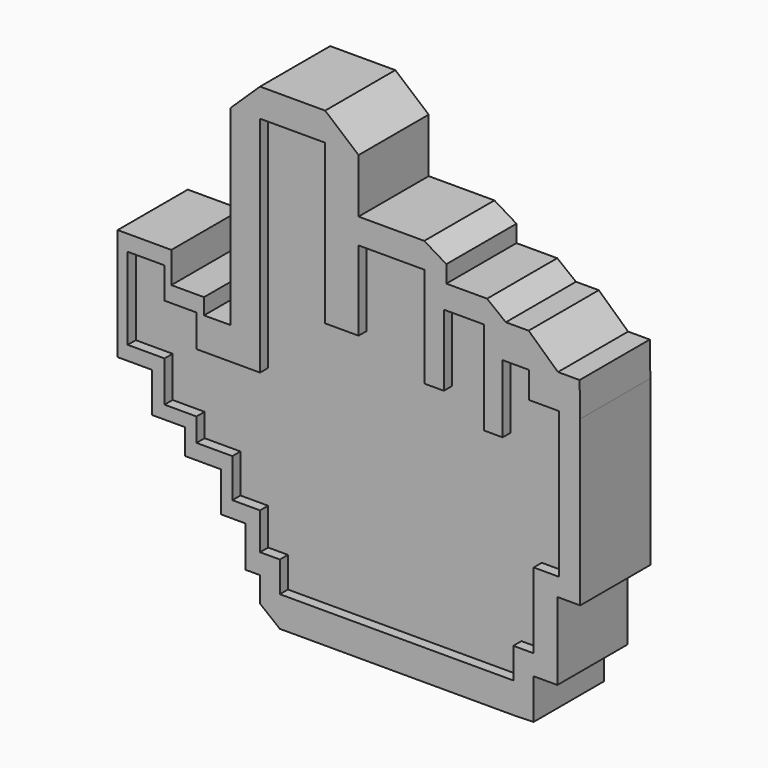
from build123d import *

# Parameters (mm, degrees)
F1_DEPTH = 11.684
F2_DEPTH = 13.208


# Not quite as in the source:
# - a feature names something its author has since deleted; it is built from what else it names


with BuildPart() as f1:
    # F0 (on Front) → F1 (new body)
    with BuildSketch(Plane.XZ):
        Polygon((9.8076034337, -4.2564473115), (0, -4.2564473115), (0, -28.2072033733), (0, -37.9272252321), (-4.4246674515, -37.9272252321), (-9.569064714, -37.9272252321), (-9.569064714, -33.0672143027), (-14.3852122128, -33.0672143027), (-14.3852122128, -28.3846426755), (-19.9310798198, -28.3846426755), (-19.9310798198, -40.7246947289), (-14.3852122128, -40.7246947289), (-14.3852122128, -46.85433954), (-9.569064714, -46.85433954), (-9.569064714, -50.3569915891), (-4.1691423394, -50.3569915891), (-4.1691423394, -56.1947450042), (0, -56.1947450042), (0, -61.7406144738), (2.9821074568, -61.7406144738), (2.9821074568, -66.3378462195), (38.154579699, -66.3378462195), (38.154579699, -61.7406144738), (41.2194021046, -61.7406144738), (41.2194021046, -50.3569915891), (45.0411513448, -50.3569915891), (45.0411513448, -28.3846426755), (40.5284799635, -28.3846426755), (40.5284799635, -24.3923105299), (36.5364998579, -24.3923105299), (36.5364998579, -34.6322879195), (33.7594784796, -34.6322879195), (33.7594784796, -24.3923105299), (33.7594784796, -20.5733645707), (27.6847239584, -20.5733645707), (27.6847239584, -31.3338786364), (24.7341338545, -31.3338786364), (24.7341338545, -20.5733645707), (24.7341338545, -16.2325797137), (14.8409679532, -16.2325797137), (14.8409679532, -28.2087121159), (9.8076034337, -28.2087121159), align=None)
    extrude(amount=F1_DEPTH)

    # F0 (on Front) → F2 (join)
    with BuildSketch(Plane.XZ):
        Polygon((9.8076034337, 0), (0, 0), (-4.4246674515, -4.2564473115), (-4.4246674515, -28.2072033733), (-4.4246674515, -33.0672143027), (-8.441273123, -33.0877043307), (-8.441273123, -30.6703820825), (-13.3577445522, -30.6703820825), (-13.3577445522, -26.0001793504), (-21.4487463236, -26.0001793504), (-21.4487463236, -42.8537763655), (-16.2677373737, -42.8537763655), (-16.2677373737, -48.8393343985), (-11.3371098414, -48.8393343985), (-11.3371098414, -52.6647716761), (-5.9138466604, -52.6647716761), (-5.9138466604, -58.6375892162), (-2.1712374873, -58.6375892162), (-2.1712374873, -64.7857561707), (0, -64.7857561707), (0, -68.5636028647), (2.9821074568, -70.9350779653), (38.154579699, -70.9350779653), (41.2194021046, -70.8393231034), (41.2194021046, -64.7857561707), (44.7839312255, -64.7857561707), (44.7839312255, -61.7406144738), (44.7839312255, -53.1140379608), (48.2247062027, -53.1140379608), (48.2247062027, -50.3569915891), (48.2247062027, -28.3846426755), (48.131018877, -23.2601258904), (44.8739007115, -23.2601258904), (40.4558517039, -19.210241735), (37.0195880532, -19.210241735), (34.1969430447, -17.0012172312), (28.0607584864, -17.0012172312), (28.0607584864, -14.4240194932), (24.7341338545, -12.4151380733), (14.8409679532, -12.4151380733), (14.8409679532, -4.2564473115), align=None)
        Polygon((0, -28.2072033733), (0, -4.2564473115), (9.8076034337, -4.2564473115), (9.8076034337, -28.2087121159), (14.8409679532, -28.2087121159), (14.8409679532, -16.2325797137), (24.7341338545, -16.2325797137), (24.7341338545, -20.5733645707), (24.7341338545, -31.3338786364), (27.6847239584, -31.3338786364), (27.6847239584, -20.5733645707), (33.7594784796, -20.5733645707), (33.7594784796, -24.3923105299), (33.7594784796, -34.6322879195), (36.5364998579, -34.6322879195), (36.5364998579, -24.3923105299), (40.5284799635, -24.3923105299), (40.5284799635, -28.3846426755), (45.0411513448, -28.3846426755), (45.0411513448, -50.3569915891), (41.2194021046, -50.3569915891), (41.2194021046, -61.7406144738), (38.154579699, -61.7406144738), (38.154579699, -66.3378462195), (2.9821074568, -66.3378462195), (2.9821074568, -61.7406144738), (0, -61.7406144738), (0, -56.1947450042), (-4.1691423394, -56.1947450042), (-4.1691423394, -50.3569915891), (-9.569064714, -50.3569915891), (-9.569064714, -46.85433954), (-14.3852122128, -46.85433954), (-14.3852122128, -40.7246947289), (-19.9310798198, -40.7246947289), (-19.9310798198, -28.3846426755), (-14.3852122128, -28.3846426755), (-14.3852122128, -33.0672143027), (-9.569064714, -33.0672143027), (-9.569064714, -37.9272252321), (-4.4246674515, -37.9272252321), (0, -37.9272252321), align=None, mode=Mode.SUBTRACT)
    extrude(amount=F2_DEPTH)


solid = f1.part
